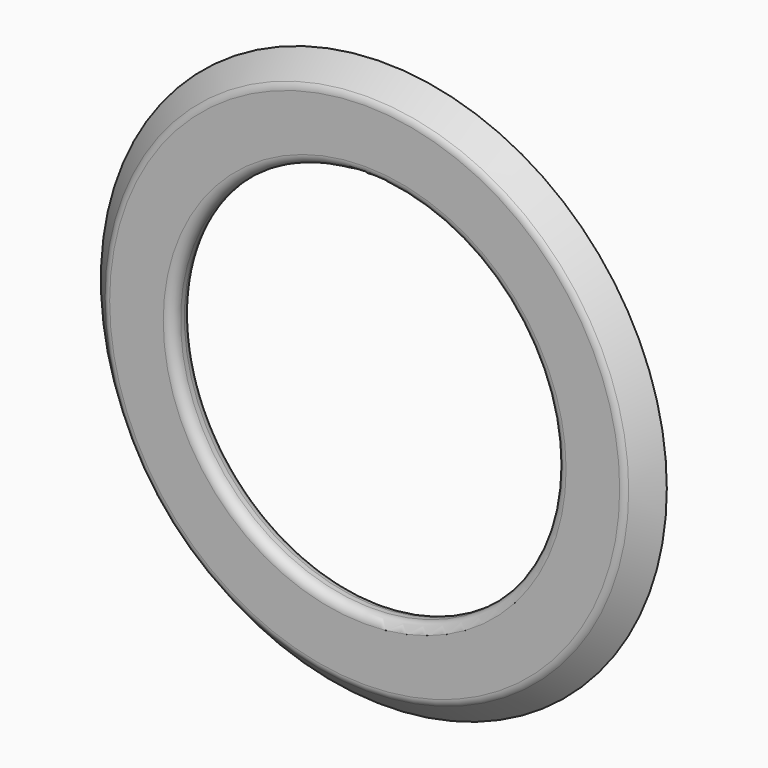
from build123d import *

# Parameters (mm, degrees)
F0_R     = 38.1
F0_R_2   = 25.4
F1_DEPTH = 3.175
F2_R     = 1.27
F3_R     = 1.27


# Not quite as in the source:
# - a fillet or chamfer that OpenCascade refuses, or shapes differently, is made with other operations: its cross-section is extruded or revolved along the edge and cut away or added


with BuildPart() as f1:
    # F0 (on Front) → F1 (new body)
    with BuildSketch(Plane.XZ):
        Circle(F0_R)
        Circle(F0_R_2, mode=Mode.SUBTRACT)
    extrude(amount=F1_DEPTH)

    # F2
    f2_edges = [f1.edges().sort_by_distance(p)[0] for p in [
        (-25.4, 0, 0),
        (-25.4, -3.175, 0),
    ]]
    fillet(f2_edges, radius=F2_R)

    # F4: chamfer of 3.81 on 1 edges, made by hand

    # F4_s1 → F4_t2 (revolve, cut)
    with BuildSketch(Plane.XY):
        Polygon((34.29, -3.175), (38.1, 0.635), (38.1, -3.175), align=None)
    revolve(axis=Axis((0, -3.175, 0), (0, -1, 0)), mode=Mode.SUBTRACT)

    # F3
    f3_edges = [f1.edges().sort_by_distance(p)[0] for p in [
        (-34.29, -3.175, 0),
    ]]
    fillet(f3_edges, radius=F3_R)


solid = f1.part
